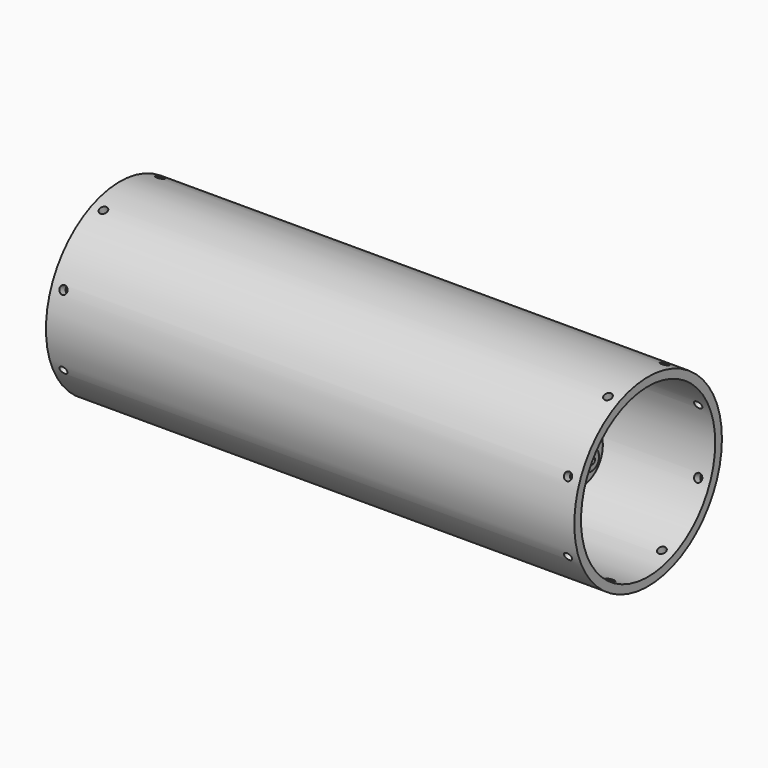
from build123d import *

# Parameters (mm, degrees)
F5_D             = 5
F5_DEPTH         = 10
F5_TIP           = 1.5021515476
F5_ON_F3_D       = 5
F5_ON_F3_DEPTH   = 10
F5_ON_F3_TIP     = 1.5021515476
F6_R             = 3.15
F7_DEPTH         = 1.6
F9_DEPTH         = 25
F10_R            = 0.8
F11_R            = 3.25
F12_DEPTH        = 1.6
F16_DEPTH        = 25
F17_R            = 69.85
F17_R_2          = 63.5
F18_DEPTH        = 125
F18_DEPTH_BACK   = 275
F21_DEPTH        = 180
F24_R            = 1
F27_D            = 6.6
F27_DEPTH        = 12
F27_TIP          = 1.9828400428
F27_ON_F25_D     = 6.6
F27_ON_F25_DEPTH = 12
F27_ON_F25_TIP   = 1.9828400428
F29_D            = 2.5
F29_DEPTH        = 13.5
F29_TIP          = 0.7510757738
F31_DEPTH        = 10
F34_SIZE         = 1
F35_SIZE         = 0.25
F36_R            = 0.2
F37_SIZE2        = 0.3526539614
F37_SIZE         = 2
F38_SIZE2        = 0.3526539614
F38_SIZE         = 2
F39_SIZE         = 1
F42_D            = 2.5
F42_DEPTH        = 6
F42_TIP          = 0.7510757738
F42_ON_F41_D     = 2.5
F42_ON_F41_DEPTH = 6
F42_ON_F41_TIP   = 0.7510757738
F44_D            = 2.5
F44_DEPTH        = 12
F44_TIP          = 0.7510757738
F65_D            = 6
F65_DEPTH        = 12
F65_START        = 0.0644536
F65_TIP          = 1.8025818571
F65_ON_F64_D     = 6
F65_ON_F64_DEPTH = 12
F65_ON_F64_START = 0.0644536
F65_ON_F64_TIP   = 1.8025818571
F65_ON_F63_D     = 6
F65_ON_F63_DEPTH = 12
F65_ON_F63_START = 0.0644536
F65_ON_F63_TIP   = 1.8025818571
F65_ON_F62_D     = 6
F65_ON_F62_DEPTH = 12
F65_ON_F62_START = 0.0644536
F65_ON_F62_TIP   = 1.8025818571
F65_ON_F61_D     = 6
F65_ON_F61_DEPTH = 12
F65_ON_F61_START = 0.0644536
F65_ON_F61_TIP   = 1.8025818571
F65_ON_F60_D     = 6
F65_ON_F60_DEPTH = 12
F65_ON_F60_START = 0.0644536
F65_ON_F60_TIP   = 1.8025818571
F65_ON_F59_D     = 6
F65_ON_F59_DEPTH = 12
F65_ON_F59_START = 0.0644536
F65_ON_F59_TIP   = 1.8025818571
F65_ON_F57_D     = 6
F65_ON_F57_DEPTH = 12
F65_ON_F57_START = 0.0644536
F65_ON_F57_TIP   = 1.8025818571


# Not quite as in the source:
# - a fillet or chamfer that OpenCascade refuses, or shapes differently, is made with other operations: its cross-section is extruded or revolved along the edge and cut away or added
# - a length typed as a fraction of an inch, garbled in the dataset ("3 / 203.2 mm" for 3/8 in), is restored
# - a feature names something its author has since deleted; it is built from what else it names


with BuildPart() as f1:
    # F0 (on Front) → F1 (revolve)
    with BuildSketch(Plane.XZ):
        Polygon((-82.75, 6.75), (-82.75, 0), (82.75, 0), (82.75, 7.75), (75.5, 7.75), (75.5, 20.325), (-75.5, 20.325), (-75.5, 12.8), (-80.8795903936, 12.8), (-80.8795903936, 6.75), align=None)
    revolve(axis=Axis((0, 0, 0), (1, 0, 0)))

    # F2: fillet of radius 2 on 6 edges, made by hand

    # F2_s1 → F2_t2 (revolve, cut)
    with BuildSketch(Plane.XZ):
        with BuildLine():
            ThreePointArc((75.5, 18.325), (74.9142135624, 19.7392135624), (73.5, 20.325))
            Line((73.5, 20.325), (75.5, 20.325))
            Line((75.5, 20.325), (75.5, 18.325))
        make_face()
    revolve(axis=Axis((75.5, 0, 0), (1, 0, 0)), mode=Mode.SUBTRACT)

    # F2_s3 → F2_t4 (revolve, cut)
    with BuildSketch(Plane.XZ):
        with BuildLine():
            ThreePointArc((-73.5, 20.325), (-74.9142135624, 19.7392135624), (-75.5, 18.325))
            Line((-75.5, 18.325), (-75.5, 20.325))
            Line((-75.5, 20.325), (-73.5, 20.325))
        make_face()
    revolve(axis=Axis((-75.5, 0, 0), (1, 0, 0)), mode=Mode.SUBTRACT)

    # F2_s5 → F2_t6 (revolve, cut)
    with BuildSketch(Plane.XZ):
        with BuildLine():
            ThreePointArc((82.75, 5.75), (82.1642135624, 7.1642135624), (80.75, 7.75))
            Line((80.75, 7.75), (82.75, 7.75))
            Line((82.75, 7.75), (82.75, 5.75))
        make_face()
    revolve(axis=Axis((82.75, 0, 0), (1, 0, 0)), mode=Mode.SUBTRACT)

    # F2_s7 → F2_t8 (revolve, cut)
    with BuildSketch(Plane.XZ):
        with BuildLine():
            ThreePointArc((-78.8795903936, 12.8), (-80.293803956, 12.2142135624), (-80.8795903936, 10.8))
            Line((-80.8795903936, 10.8), (-80.8795903936, 12.8))
            Line((-80.8795903936, 12.8), (-78.8795903936, 12.8))
        make_face()
    revolve(axis=Axis((-80.8795903936, 0, 0), (1, 0, 0)), mode=Mode.SUBTRACT)

    # F2_s9 → F2_t10 (revolve, cut)
    with BuildSketch(Plane.XZ):
        with BuildLine():
            ThreePointArc((-82.75, 4.7542028335), (-82.2093116164, 6.1218320253), (-80.8795903936, 6.75))
            Line((-80.8795903936, 6.75), (-82.75, 6.75))
            Line((-82.75, 6.75), (-82.75, 4.7542028335))
        make_face()
    revolve(axis=Axis((-82.75, 0, 0), (1, 0, 0)), mode=Mode.SUBTRACT)

    # F5
    with Locations(Plane.YZ.offset(82.75)):
        with Locations((0, 0)):
            Hole(F5_D / 2, depth=F5_DEPTH)
            with Locations((0, 0, -(F5_DEPTH + F5_TIP / 2))):  # 118° drill point
                Cone(0, F5_D / 2, F5_TIP, mode=Mode.SUBTRACT)

    # F5 on F3
    with Locations(Plane(origin=(-82.75, 0, 0), x_dir=(0, -1, 0), z_dir=(-1, 0, 0))):
        with Locations((0, 0)):
            Hole(F5_ON_F3_D / 2, depth=F5_ON_F3_DEPTH)
            with Locations((0, 0, -(F5_ON_F3_DEPTH + F5_ON_F3_TIP / 2))):  # 118° drill point
                Cone(0, F5_ON_F3_D / 2, F5_ON_F3_TIP, mode=Mode.SUBTRACT)


with BuildPart() as f7:
    # F6 (on face) → F7 (new body)
    with BuildSketch(Plane(origin=(-82.75, 0, 0), x_dir=(0, -1, 0), z_dir=(-1, 0, 0))):
        with BuildLine():
            ThreePointArc((0, 63), (-44.5477272148, -44.5477272148), (63, 0))
            ThreePointArc((63, 0), (60.8533270562, 16.3055998415), (54.5596004384, 31.5))
            ThreePointArc((54.5596004384, 31.5), (41.4538346793, 41.4035652394), (25.2189816103, 38.8993195624))
            Line((25.2189816103, 38.8993195624), (21.0783081258, 41.2899385133))
            ThreePointArc((21.0783081258, 41.2899385133), (18.1007232385, 52.7313018973), (9.4337941097, 60.7721443483))
            ThreePointArc((9.4337941097, 60.7721443483), (4.8466434805, 62.4354798817), (0, 63))
        make_face()
        with Locations((-36.2972897361, -20.95625)):
            Circle(F6_R, mode=Mode.SUBTRACT)
        with Locations((0, -41.9125)):
            Circle(F6_R, mode=Mode.SUBTRACT)
        with Locations((36.2972897361, -20.95625)):
            Circle(F6_R, mode=Mode.SUBTRACT)
        with Locations((-36.2972897361, 20.95625)):
            Circle(F6_R, mode=Mode.SUBTRACT)
        Circle(F6_R, mode=Mode.SUBTRACT)
        with Locations((36.2972897361, 20.95625)):
            Circle(F6_R, mode=Mode.SUBTRACT)
        with Locations((0, 41.9125)):
            Circle(F6_R, mode=Mode.SUBTRACT)
        with BuildLine():
            ThreePointArc((25.2189816103, 38.8993195624), (41.4538346793, 41.4035652394), (54.5596004384, 31.5))
            ThreePointArc((54.5596004384, 31.5), (35.6036827691, 51.9747801657), (9.6638866489, 62.2543917715))
            Line((9.6638866489, 62.2543917715), (9.4337941097, 60.7721443483))
            ThreePointArc((9.4337941097, 60.7721443483), (18.1007232385, 52.7313018973), (21.0783081258, 41.2899385133))
            Line((21.0783081258, 41.2899385133), (25.2189816103, 38.8993195624))
        make_face()
        with BuildLine():
            ThreePointArc((9.6638866489, 62.2543917715), (4.8463036635, 62.8133213642), (0, 63))
            ThreePointArc((0, 63), (4.8466434805, 62.4354798817), (9.4337941097, 60.7721443483))
            Line((9.4337941097, 60.7721443483), (9.6638866489, 62.2543917715))
        make_face()
    extrude(amount=F7_DEPTH)

    # F8 (on face) → F9 (cut)
    with BuildSketch(Plane(origin=(-84.35, 0, 0), x_dir=(0, -1, 0), z_dir=(-1, 0, 0))):
        with BuildLine():
            ThreePointArc((9.5220951433, 61.3409762624), (9.5968863226, 60.8608876958), (9.9356949866, 60.5126242303))
            ThreePointArc((9.9356949866, 60.5126242303), (18.1268267596, 52.6875084862), (21.0868962348, 41.7529273405))
            ThreePointArc((21.0868962348, 41.7529273405), (21.1925445213, 41.3494978318), (21.4868733296, 41.0540532829))
            Line((21.4868733296, 41.0540532829), (24.8104164065, 39.1352047928))
            ThreePointArc((24.8104164065, 39.1352047928), (25.2134432954, 39.0280308421), (25.6156476418, 39.1382514965))
            ThreePointArc((25.6156476418, 39.1382514965), (36.5653074314, 42.0420467069), (47.4376223398, 38.8608763778))
            ThreePointArc((47.4376223398, 38.8608763778), (47.9086316802, 38.7415912005), (48.3617961645, 38.9168644225))
            Line((48.3617961645, 38.9168644225), (49.0819414468, 39.496367223))
            ThreePointArc((49.0819414468, 39.496367223), (31.5, 54.5596004384), (9.6638866489, 62.2543917715))
            Line((9.6638866489, 62.2543917715), (9.5220951433, 61.3409762624))
        make_face()
        with BuildLine():
            ThreePointArc((-48.3617961645, 38.9168644225), (-47.9086316802, 38.7415912005), (-47.4376223398, 38.8608763778))
            ThreePointArc((-47.4376223398, 38.8608763778), (-36.5653074314, 42.0420467069), (-25.6156476418, 39.1382514965))
            ThreePointArc((-25.6156476418, 39.1382514965), (-25.2134432954, 39.0280308421), (-24.8104164065, 39.1352047928))
            Line((-24.8104164065, 39.1352047928), (-21.4868733296, 41.0540532829))
            ThreePointArc((-21.4868733296, 41.0540532829), (-21.1925445213, 41.3494978318), (-21.0868962348, 41.7529273405))
            ThreePointArc((-21.0868962348, 41.7529273405), (-18.1268267596, 52.6875084862), (-9.9356949866, 60.5126242303))
            ThreePointArc((-9.9356949866, 60.5126242303), (-9.5968863226, 60.8608876958), (-9.5220951433, 61.3409762624))
            Line((-9.5220951433, 61.3409762624), (-9.6638866489, 62.2543917715))
            ThreePointArc((-9.6638866489, 62.2543917715), (-31.5, 54.5596004384), (-49.0819414468, 39.496367223))
            Line((-49.0819414468, 39.496367223), (-48.3617961645, 38.9168644225))
        make_face()
        with BuildLine():
            ThreePointArc((-57.8838913078, -22.4241118398), (-57.5055180028, -22.1192964953), (-57.3733173264, -21.6517478525))
            ThreePointArc((-57.3733173264, -21.6517478525), (-54.692134191, -10.6454617793), (-46.7025438766, -2.614675844))
            ThreePointArc((-46.7025438766, -2.614675844), (-46.4059878167, -2.3214669896), (-46.2972897361, -1.9188484901))
            Line((-46.2972897361, -1.9188484901), (-46.2972897361, 1.9188484901))
            ThreePointArc((-46.2972897361, 1.9188484901), (-46.4059878167, 2.3214669896), (-46.7025438766, 2.614675844))
            ThreePointArc((-46.7025438766, 2.614675844), (-54.692134191, 10.6454617793), (-57.3733173264, 21.6517478525))
            ThreePointArc((-57.3733173264, 21.6517478525), (-57.5055180028, 22.1192964953), (-57.8838913078, 22.4241118398))
            Line((-57.8838913078, 22.4241118398), (-58.7458280957, 22.7580245485))
            ThreePointArc((-58.7458280957, 22.7580245485), (-63, 0), (-58.7458280957, -22.7580245485))
            Line((-58.7458280957, -22.7580245485), (-57.8838913078, -22.4241118398))
        make_face()
        with BuildLine():
            ThreePointArc((-9.5220951433, -61.3409762624), (-9.5968863226, -60.8608876958), (-9.9356949866, -60.5126242303))
            ThreePointArc((-9.9356949866, -60.5126242303), (-18.1268267596, -52.6875084862), (-21.0868962348, -41.7529273405))
            ThreePointArc((-21.0868962348, -41.7529273405), (-21.1925445213, -41.3494978318), (-21.4868733296, -41.0540532829))
            Line((-21.4868733296, -41.0540532829), (-24.8104164065, -39.1352047928))
            ThreePointArc((-24.8104164065, -39.1352047928), (-25.2134432954, -39.0280308421), (-25.6156476418, -39.1382514965))
            ThreePointArc((-25.6156476418, -39.1382514965), (-36.5653074314, -42.0420467069), (-47.4376223398, -38.8608763778))
            ThreePointArc((-47.4376223398, -38.8608763778), (-47.9086316802, -38.7415912005), (-48.3617961645, -38.9168644225))
            Line((-48.3617961645, -38.9168644225), (-49.0819414468, -39.496367223))
            ThreePointArc((-49.0819414468, -39.496367223), (-31.5, -54.5596004384), (-9.6638866489, -62.2543917715))
            Line((-9.6638866489, -62.2543917715), (-9.5220951433, -61.3409762624))
        make_face()
        with BuildLine():
            ThreePointArc((48.3617961645, -38.9168644225), (47.9086316802, -38.7415912005), (47.4376223398, -38.8608763778))
            ThreePointArc((47.4376223398, -38.8608763778), (36.5653074314, -42.0420467069), (25.6156476418, -39.1382514965))
            ThreePointArc((25.6156476418, -39.1382514965), (25.2134432954, -39.0280308421), (24.8104164065, -39.1352047928))
            Line((24.8104164065, -39.1352047928), (21.4868733296, -41.0540532829))
            ThreePointArc((21.4868733296, -41.0540532829), (21.1925445213, -41.3494978318), (21.0868962348, -41.7529273405))
            ThreePointArc((21.0868962348, -41.7529273405), (18.1268267596, -52.6875084862), (9.9356949866, -60.5126242303))
            ThreePointArc((9.9356949866, -60.5126242303), (9.5968863226, -60.8608876958), (9.5220951433, -61.3409762624))
            Line((9.5220951433, -61.3409762624), (9.6638866489, -62.2543917715))
            ThreePointArc((9.6638866489, -62.2543917715), (31.5, -54.5596004384), (49.0819414468, -39.496367223))
            Line((49.0819414468, -39.496367223), (48.3617961645, -38.9168644225))
        make_face()
        with BuildLine():
            ThreePointArc((57.8838913078, 22.4241118398), (57.5055180028, 22.1192964953), (57.3733173264, 21.6517478525))
            ThreePointArc((57.3733173264, 21.6517478525), (54.692134191, 10.6454617793), (46.7025438766, 2.614675844))
            ThreePointArc((46.7025438766, 2.614675844), (46.4059878167, 2.3214669896), (46.2972897361, 1.9188484901))
            Line((46.2972897361, 1.9188484901), (46.2972897361, -1.9188484901))
            ThreePointArc((46.2972897361, -1.9188484901), (46.4059878167, -2.3214669896), (46.7025438766, -2.614675844))
            ThreePointArc((46.7025438766, -2.614675844), (54.692134191, -10.6454617793), (57.3733173264, -21.6517478525))
            ThreePointArc((57.3733173264, -21.6517478525), (57.5055180028, -22.1192964953), (57.8838913078, -22.4241118398))
            Line((57.8838913078, -22.4241118398), (58.7458280957, -22.7580245485))
            ThreePointArc((58.7458280957, -22.7580245485), (63, 0), (58.7458280957, 22.7580245485))
            Line((58.7458280957, 22.7580245485), (57.8838913078, 22.4241118398))
        make_face()
    extrude(amount=-F9_DEPTH, mode=Mode.SUBTRACT)

    # F10
    f10_edges = [f7.edges().sort_by_distance(p)[0] for p in [
        (-83.55, -9.663887, 62.254392),
        (-83.55, -49.081941, 39.496367),
    ]]
    fillet(f10_edges, radius=F10_R)


with BuildPart() as f12:
    # F11 (on face) → F12 (new body)
    with BuildSketch(Plane(origin=(-84.35, 0, 0), x_dir=(0, -1, 0), z_dir=(-1, 0, 0))):
        with BuildLine():
            ThreePointArc((5, 50.5727540378), (-8.6602540378, 46.9125), (-5, 33.2522459622))
            Line((-5, 33.2522459622), (31.2972897361, 12.2959959622))
            ThreePointArc((31.2972897361, 12.2959959622), (44.957543774, 15.95625), (41.2972897361, 29.6165040378))
            Line((41.2972897361, 29.6165040378), (24.8104164065, 39.1352047928))
            Line((24.8104164065, 39.1352047928), (21.4868733296, 41.0540532829))
            Line((21.4868733296, 41.0540532829), (5, 50.5727540378))
        make_face()
        with Locations((36.2972897361, 20.95625)):
            Circle(F11_R, mode=Mode.SUBTRACT)
        with Locations((0, 41.9125)):
            Circle(F11_R, mode=Mode.SUBTRACT)
    extrude(amount=F12_DEPTH)


with BuildPart() as f14:
    # F13 (on Front) → F14 (revolve)
    with BuildSketch(Plane.XZ):
        with BuildLine():
            Line((-87.95, 41.9125), (-82.75, 41.9125))
            Line((-82.75, 41.9125), (-77.95, 41.9125))
            Line((-77.95, 41.9125), (-77.95, 44.9125))
            Line((-77.95, 44.9125), (-85.95, 44.9125))
            Line((-85.95, 44.9125), (-85.95, 46.9125))
            Line((-85.95, 46.9125), (-86.45, 46.9125))
            ThreePointArc((-86.45, 46.9125), (-87.5669220908, 44.5225766272), (-87.95, 41.9125))
        make_face()
    revolve(axis=Axis((-73.6735029377, 0, 41.9125), (-1, 0, 0)))

    # F15 (on face) → F16 (cut)
    with BuildSketch(Plane(origin=(-85.95, 0, 0), x_dir=(0, -1, 0), z_dir=(-1, 0, 0))):
        Polygon((0.5, 44.4125), (0, 44.4125), (-0.5, 44.4125), (-0.5, 42.4125), (-2.5, 42.4125), (-2.5, 41.9125), (-2.5, 41.4125), (-0.5, 41.4125), (-0.5, 39.4125), (0, 39.4125), (0.5, 39.4125), (0.5, 41.4125), (2.5, 41.4125), (2.5, 41.9125), (2.5, 42.4125), (0.5, 42.4125), align=None)
    extrude(amount=F16_DEPTH, mode=Mode.SUBTRACT)


with BuildPart() as f18:
    # F17 (on Right) → F18 (new body, two sides)
    with BuildSketch(Plane.YZ) as f18_sk:
        Circle(F17_R)
        Circle(F17_R_2, mode=Mode.SUBTRACT)
    extrude(amount=F18_DEPTH)
    extrude(f18_sk.sketch, amount=-F18_DEPTH_BACK)

    # F65
    # its depths count from where the whole tool has entered the part; down to there all is cleared
    with Locations(Plane(origin=(0, -26.7304377507, 64.5329853459), x_dir=(1, 0, 0), z_dir=(0, -0.3826834324, 0.9238795325)).offset(-F65_START)):
        with Locations((-266, 0), (116, 0)):
            Hole(F65_D / 2, depth=F65_DEPTH)
            with Locations((0, 0, -(F65_DEPTH + F65_TIP / 2))):  # 118° drill point
                Cone(0, F65_D / 2, F65_TIP, mode=Mode.SUBTRACT)

    # F65 on F64
    # its depths count from where the whole tool has entered the part; down to there all is cleared
    with Locations(Plane(origin=(0, 26.7304377507, 64.5329853459), x_dir=(1, 0, 0), z_dir=(0, 0.3826834324, 0.9238795325)).offset(-F65_ON_F64_START)):
        with Locations((-266, 0), (116, 0)):
            Hole(F65_ON_F64_D / 2, depth=F65_ON_F64_DEPTH)
            with Locations((0, 0, -(F65_ON_F64_DEPTH + F65_ON_F64_TIP / 2))):  # 118° drill point
                Cone(0, F65_ON_F64_D / 2, F65_ON_F64_TIP, mode=Mode.SUBTRACT)

    # F65 on F63
    # its depths count from where the whole tool has entered the part; down to there all is cleared
    with Locations(Plane(origin=(0, 64.5329853459, 26.7304377507), x_dir=(-1, 0, 0), z_dir=(0, 0.9238795325, 0.3826834324)).offset(-F65_ON_F63_START)):
        with Locations((266, 0), (-116, 0)):
            Hole(F65_ON_F63_D / 2, depth=F65_ON_F63_DEPTH)
            with Locations((0, 0, -(F65_ON_F63_DEPTH + F65_ON_F63_TIP / 2))):  # 118° drill point
                Cone(0, F65_ON_F63_D / 2, F65_ON_F63_TIP, mode=Mode.SUBTRACT)

    # F65 on F62
    # its depths count from where the whole tool has entered the part; down to there all is cleared
    with Locations(Plane(origin=(0, 64.5329853459, -26.7304377507), x_dir=(-1, 0, 0), z_dir=(0, 0.9238795325, -0.3826834324)).offset(-F65_ON_F62_START)):
        with Locations((266, 0), (-116, 0)):
            Hole(F65_ON_F62_D / 2, depth=F65_ON_F62_DEPTH)
            with Locations((0, 0, -(F65_ON_F62_DEPTH + F65_ON_F62_TIP / 2))):  # 118° drill point
                Cone(0, F65_ON_F62_D / 2, F65_ON_F62_TIP, mode=Mode.SUBTRACT)

    # F65 on F61
    # its depths count from where the whole tool has entered the part; down to there all is cleared
    with Locations(Plane(origin=(0, 26.7304377507, -64.5329853459), x_dir=(1, 0, 0), z_dir=(0, 0.3826834324, -0.9238795325)).offset(-F65_ON_F61_START)):
        with Locations((-266, 0), (116, 0)):
            Hole(F65_ON_F61_D / 2, depth=F65_ON_F61_DEPTH)
            with Locations((0, 0, -(F65_ON_F61_DEPTH + F65_ON_F61_TIP / 2))):  # 118° drill point
                Cone(0, F65_ON_F61_D / 2, F65_ON_F61_TIP, mode=Mode.SUBTRACT)

    # F65 on F60
    # its depths count from where the whole tool has entered the part; down to there all is cleared
    with Locations(Plane(origin=(0, -26.7304377507, -64.5329853459), x_dir=(1, 0, 0), z_dir=(0, -0.3826834324, -0.9238795325)).offset(-F65_ON_F60_START)):
        with Locations((-266, 0), (116, 0)):
            Hole(F65_ON_F60_D / 2, depth=F65_ON_F60_DEPTH)
            with Locations((0, 0, -(F65_ON_F60_DEPTH + F65_ON_F60_TIP / 2))):  # 118° drill point
                Cone(0, F65_ON_F60_D / 2, F65_ON_F60_TIP, mode=Mode.SUBTRACT)

    # F65 on F59
    # its depths count from where the whole tool has entered the part; down to there all is cleared
    with Locations(Plane(origin=(0, -64.5329853459, -26.7304377507), x_dir=(1, 0, 0), z_dir=(0, -0.9238795325, -0.3826834324)).offset(-F65_ON_F59_START)):
        with Locations((-266, 0), (116, 0)):
            Hole(F65_ON_F59_D / 2, depth=F65_ON_F59_DEPTH)
            with Locations((0, 0, -(F65_ON_F59_DEPTH + F65_ON_F59_TIP / 2))):  # 118° drill point
                Cone(0, F65_ON_F59_D / 2, F65_ON_F59_TIP, mode=Mode.SUBTRACT)

    # F65 on F57
    # its depths count from where the whole tool has entered the part; down to there all is cleared
    with Locations(Plane(origin=(0, -64.5329853459, 26.7304377507), x_dir=(1, 0, 0), z_dir=(0, -0.9238795325, 0.3826834324)).offset(-F65_ON_F57_START)):
        with Locations((-266, 0), (116, 0)):
            Hole(F65_ON_F57_D / 2, depth=F65_ON_F57_DEPTH)
            with Locations((0, 0, -(F65_ON_F57_DEPTH + F65_ON_F57_TIP / 2))):  # 118° drill point
                Cone(0, F65_ON_F57_D / 2, F65_ON_F57_TIP, mode=Mode.SUBTRACT)


with BuildPart() as f21:
    # F20 (on offset) → F21 (new body)
    with BuildSketch(Plane.YZ.offset(90.9875)):
        Polygon((-25.7679491924, 50.6313972081), (-29.2320508076, 50.6313972081), (-30.9641016151, 47.6313972081), (-29.2320508076, 44.6313972081), (-25.7679491924, 44.6313972081), (-24.0358983849, 47.6313972081), align=None)
    extrude(amount=-F21_DEPTH)

    # F29
    with Locations(Plane.YZ.offset(90.9875)):
        with Locations((-27.5, 47.6313972081)):
            Hole(F29_D / 2, depth=F29_DEPTH)
            with Locations((0, 0, -(F29_DEPTH + F29_TIP / 2))):  # 118° drill point
                Cone(0, F29_D / 2, F29_TIP, mode=Mode.SUBTRACT)

    # F30 (on face) → F31 (cut)
    with BuildSketch(Plane.YZ.offset(90.9875)):
        with BuildLine():
            ThreePointArc((-27.5, 50.6313972081), (-25.9999998915, 50.2294733569), (-24.9019236634, 49.1313969912))
            Line((-24.9019236634, 49.1313969912), (-25.7679491924, 50.6313972081))
            Line((-25.7679491924, 50.6313972081), (-27.5, 50.6313972081))
        make_face()
        with BuildLine():
            ThreePointArc((-30.0980762129, 49.1313972054), (-29.0000000014, 50.2294734187), (-27.5, 50.6313972081))
            Line((-27.5, 50.6313972081), (-29.2320508076, 50.6313972081))
            Line((-29.2320508076, 50.6313972081), (-30.0980762129, 49.1313972054))
        make_face()
        with BuildLine():
            ThreePointArc((-30.0980762365, 46.1313972518), (-30.5, 47.6313972318), (-30.0980762129, 49.1313972054))
            Line((-30.0980762129, 49.1313972054), (-30.9641016151, 47.6313972081))
            Line((-30.9641016151, 47.6313972081), (-30.0980762365, 46.1313972518))
        make_face()
        with BuildLine():
            Line((-29.2320508076, 44.6313972081), (-27.5, 44.6313972081))
            ThreePointArc((-27.5, 44.6313972081), (-29.0000000218, 45.0333210094), (-30.0980762365, 46.1313972518))
            Line((-30.0980762365, 46.1313972518), (-29.2320508076, 44.6313972081))
        make_face()
        with BuildLine():
            Line((-25.7679491924, 44.6313972081), (-24.9019239254, 46.1313969714))
            ThreePointArc((-24.9019239254, 46.1313969714), (-26.0000001184, 45.0333209284), (-27.5, 44.6313972081))
            Line((-27.5, 44.6313972081), (-25.7679491924, 44.6313972081))
        make_face()
        with BuildLine():
            ThreePointArc((-24.9019236634, 49.1313969912), (-24.6022224887, 48.4078542225), (-24.5, 47.6313972081))
            ThreePointArc((-24.5, 47.6313972081), (-24.6022225565, 46.8549399408), (-24.9019239254, 46.1313969714))
            Line((-24.9019239254, 46.1313969714), (-24.0358983849, 47.6313972081))
            Line((-24.0358983849, 47.6313972081), (-24.9019236634, 49.1313969912))
        make_face()
    extrude(amount=-F31_DEPTH, mode=Mode.SUBTRACT)

    # F44
    with Locations(Plane(origin=(-89.0125, 0, 0), x_dir=(0, -1, 0), z_dir=(-1, 0, 0))):
        with Locations((27.5, 47.6313972081)):
            Hole(F44_D / 2, depth=F44_DEPTH)
            with Locations((0, 0, -(F44_DEPTH + F44_TIP / 2))):  # 118° drill point
                Cone(0, F44_D / 2, F44_TIP, mode=Mode.SUBTRACT)


with BuildPart() as f23:
    # F22 (on Front) → F23 (revolve)
    with BuildSketch(Plane.XZ):
        Polygon((-82.75, -35.1625), (-82.75, -41.9125), (51.75, -41.9125), (51.75, -34.1625), (44.5, -34.1625), (44.5, -22.9125), (-75.5, -22.9125), (-75.5, -29.1125), (-80.8795903936, -29.1125), (-80.8795903936, -35.1625), align=None)
    revolve(axis=Axis((-15.5, 0, -41.9125), (1, 0, 0)))

    # F24
    f24_edges = [f23.edges().sort_by_distance(p)[0] for p in [
        (44.5, 0, -60.9125),
        (51.75, 0, -49.6625),
        (-75.5, 0, -60.9125),
        (-80.87959, 0, -54.7125),
        (-82.75, 0, -48.6625),
    ]]
    fillet(f24_edges, radius=F24_R)

    # F27
    with Locations(Plane(origin=(-82.75, 0, 0), x_dir=(0, -1, 0), z_dir=(-1, 0, 0))):
        with Locations((0, -41.9125)):
            Hole(F27_D / 2, depth=F27_DEPTH)
            with Locations((0, 0, -(F27_DEPTH + F27_TIP / 2))):  # 118° drill point
                Cone(0, F27_D / 2, F27_TIP, mode=Mode.SUBTRACT)

    # F27 on F25
    with Locations(Plane.YZ.offset(51.75)):
        with Locations((0, -41.9125)):
            Hole(F27_ON_F25_D / 2, depth=F27_ON_F25_DEPTH)
            with Locations((0, 0, -(F27_ON_F25_DEPTH + F27_ON_F25_TIP / 2))):  # 118° drill point
                Cone(0, F27_ON_F25_D / 2, F27_ON_F25_TIP, mode=Mode.SUBTRACT)


with BuildPart() as f33:
    # F32 (on Front) → F33 (revolve)
    with BuildSketch(Plane.XZ):
        Polygon((-157.819898963, 62.992), (-158.819898963, 62.992), (-159.819898963, 62.992), (-159.819898963, 60.833), (-165.356898963, 60.833), (-165.356898963, 62.992), (-168.069898963, 62.992), (-168.069898963, 48), (-160.319898963, 48), (-160.319898963, 0), (-158.819898963, 0), (-157.319898963, 0), (-157.319898963, 48), (-149.569898963, 48), (-149.569898963, 62.992), (-152.282898963, 62.992), (-152.282898963, 60.833), (-157.819898963, 60.833), align=None)
    revolve(axis=Axis((-119.4819115173, 0, 0), (-1, 0, 0)))

    # F34
    f34_edges = [f33.edges().sort_by_distance(p)[0] for p in [
        (-168.069899, 0, -48),
        (-149.569899, 0, -48),
    ]]
    chamfer(f34_edges, length=F34_SIZE)

    # F35
    f35_edges = [f33.edges().sort_by_distance(p)[0] for p in [
        (-152.282899, 0, -62.992),
        (-157.819899, 0, -62.992),
        (-159.819899, 0, -62.992),
        (-165.356899, 0, -62.992),
    ]]
    chamfer(f35_edges, length=F35_SIZE)

    # F36
    f36_edges = [f33.edges().sort_by_distance(p)[0] for p in [
        (-152.282899, 0, -60.833),
        (-157.819899, 0, -60.833),
        (-155.051399, 0, 60.833),
        (-159.819899, 0, -60.833),
        (-165.356899, 0, -60.833),
        (-162.588399, 0, 60.833),
    ]]
    fillet(f36_edges, radius=F36_R)

    # F37
    f37_edges = [f33.edges().sort_by_distance(p)[0] for p in [
        (-168.069899, 0, -62.992),
    ]]
    chamfer(f37_edges, length=F37_SIZE, length2=F37_SIZE2)

    # F38
    f38_edges = [f33.edges().sort_by_distance(p)[0] for p in [
        (-149.569899, 0, -62.992),
    ]]
    chamfer(f38_edges, length=F38_SIZE, length2=F38_SIZE2)

    # F39
    f39_edges = [f33.edges().sort_by_distance(p)[0] for p in [
        (-160.319899, 0, -48),
        (-157.319899, 0, -48),
    ]]
    chamfer(f39_edges, length=F39_SIZE)

    # F42
    with Locations(Plane(origin=(-168.069898963, 0, 0), x_dir=(0, -1, 0), z_dir=(-1, 0, 0))):
        with Locations((-51.5, 0), (-25.75, 44.6003082949), (25.75, 44.6003082949), (51.5, 0), (25.75, -44.6003082949), (-25.75, -44.6003082949)):
            Hole(F42_D / 2, depth=F42_DEPTH)
            with Locations((0, 0, -(F42_DEPTH + F42_TIP / 2))):  # 118° drill point
                Cone(0, F42_D / 2, F42_TIP, mode=Mode.SUBTRACT)

    # F42 on F41
    with Locations(Plane.YZ.offset(-149.569898963)):
        with Locations((-25.75, 44.6003082949), (-51.5, 0), (-25.75, -44.6003082949), (25.75, -44.6003082949), (51.5, 0), (25.75, 44.6003082949)):
            Hole(F42_ON_F41_D / 2, depth=F42_ON_F41_DEPTH)
            with Locations((0, 0, -(F42_ON_F41_DEPTH + F42_ON_F41_TIP / 2))):  # 118° drill point
                Cone(0, F42_ON_F41_D / 2, F42_ON_F41_TIP, mode=Mode.SUBTRACT)


solid = Compound([f1.part, f7.part, f12.part, f14.part, f18.part, f21.part, f23.part, f33.part])
